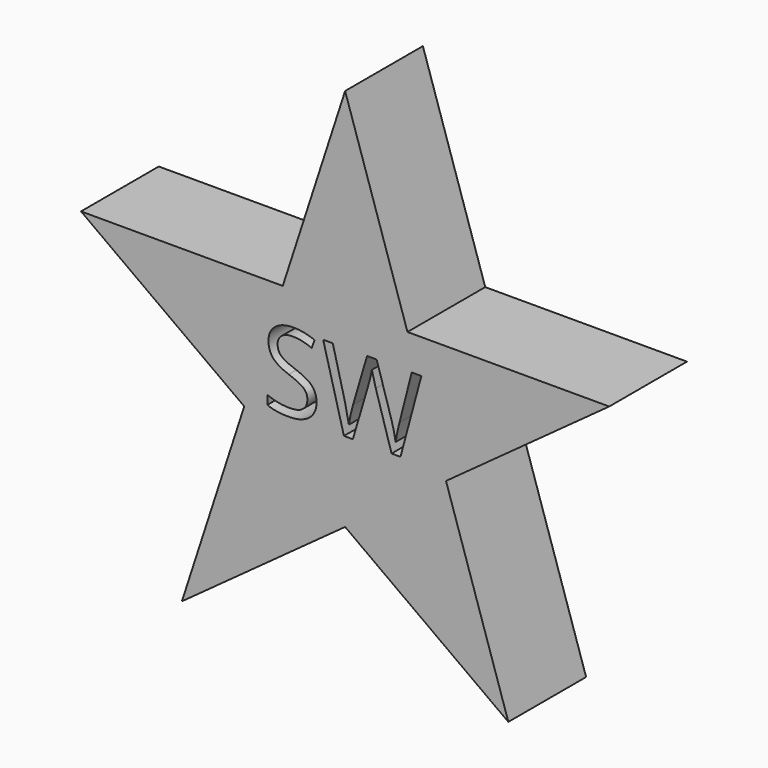
from build123d import *

# Parameters (mm, degrees)
F2_DEPTH     = 8.89
F1_TEXT_SIZE = 9.9873028876
F3_DEPTH     = 40.386


# Not quite as in the source:
# - Text() gives the source's letters only with a copy of the font that has no kerning and outlines rounded to 1/6400 em; it was checked with that copy


with BuildPart() as f2:
    # F0 (on Front) → F2 (new body)
    with BuildSketch(Plane.XZ):
        Polygon((5.7026553026, 7.8490316571), (0, 25.4), (-5.7026553026, 7.8490316571), align=None)
        Polygon((-9.2270901057, -2.9980633142), (-5.7026553026, 7.8490316571), (-24.1568355139, 7.8490316571), align=None)
        Polygon((5.7026553026, 7.8490316571), (-5.7026553026, 7.8490316571), (-9.2270901057, -2.9980633142), (0, -9.7019366858), (9.2270901057, -2.9980633142), align=None)
        Polygon((24.1568355139, 7.8490316571), (5.7026553026, 7.8490316571), (9.2270901057, -2.9980633142), align=None)
        Polygon((0, -9.7019366858), (-9.2270901057, -2.9980633142), (-14.9297454082, -20.5490316571), align=None)
        Polygon((14.9297454082, -20.5490316571), (9.2270901057, -2.9980633142), (0, -9.7019366858), align=None)
    extrude(amount=F2_DEPTH)

    # F1 (on face) → F3 (cut)
    with BuildSketch(Plane.XZ):
        with Locations((-7.62, -2.4128380418)):
            Text('SW', F1_TEXT_SIZE, font='Open Sans', text_align=(TextAlign.LEFT, TextAlign.BOTTOM))
    extrude(amount=F3_DEPTH, mode=Mode.SUBTRACT)


solid = f2.part
